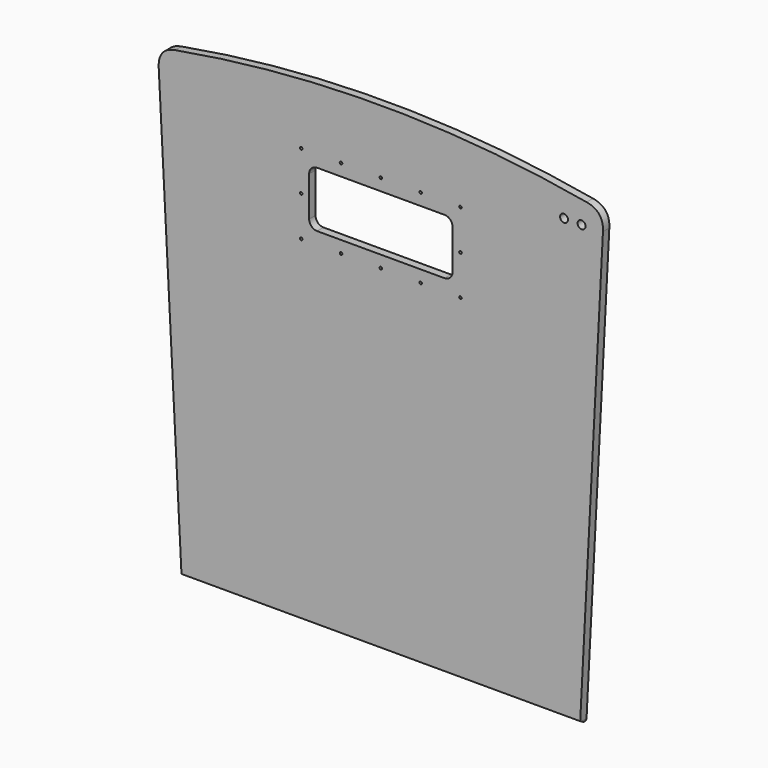
from build123d import *

# Parameters (mm, degrees)
F1_DEPTH    = 10
F2_W        = 180
F2_H        = 70
F3_DEPTH    = 10.001
F4_T1_DEPTH = 120.3455223822
F5_R        = 5
F6_T1_DEPTH = 541.5885597996
F7_R        = 10
F9_D        = 3.2
F9_DEPTH    = 6
F9_TIP      = 0.9613769904
F11_D       = 10


# Not quite as in the source:
# - a fillet or chamfer that OpenCascade refuses, or shapes differently, is made with other operations: its cross-section is extruded or revolved along the edge and cut away or added


with BuildPart() as f1:
    # F0 (on Front) → F1 (new body)
    with BuildSketch(Plane.XZ):
        with BuildLine():
            Line((-30, 578), (0, 0))
            Line((0, 0), (500, 0))
            Line((500, 0), (530, 578))
            ThreePointArc((530, 578), (250, 605), (-30, 578))
        make_face()
    extrude(amount=F1_DEPTH)

    # F2 (on face) → F3 (cut, through all)
    with BuildSketch(Plane.XZ.offset(10)):
        with Locations((250, 475)):
            Rectangle(F2_W, F2_H)
    extrude(amount=-F3_DEPTH, mode=Mode.SUBTRACT)

    # F4: fillet of radius 25 on 2 edges, made by hand

    # F4_s2 → F4_t1 (cut)
    with BuildSketch(Plane.XZ.offset(-55.1727611911)):
        with BuildLine():
            add(Edge.make_bspline(
                [(-28.865884536, 556.1493753933), (-30.0086821523, 578.1672761351), (-8.3063912994, 582.0537283993)],
                knots=[0, 0, 0, 1, 1, 1], degree=2, weights=[1, 1, 1]))
            ThreePointArc((-8.3063912994, 582.0537283993), (-19.1608272147, 580.0677046728), (-30, 578))
            Line((-30, 578), (-28.865884536, 556.1493753933))
        make_face()
        with BuildLine():
            add(Edge.make_bspline(
                [(508.3063912994, 582.0537283993), (530.0086821523, 578.1672761351), (528.865884536, 556.1493753933)],
                knots=[0, 0, 0, 1, 1, 1], degree=2, weights=[1, 1, 1]))
            Line((528.865884536, 556.1493753933), (530, 578))
            ThreePointArc((530, 578), (519.1608272147, 580.0677046728), (508.3063912994, 582.0537283993))
        make_face()
    extrude(amount=F4_T1_DEPTH, mode=Mode.SUBTRACT)

    # F5
    f5_edges = [f1.edges().sort_by_distance(p)[0] for p in [
        (500, -5, 0),
        (0, -5, 0),
    ]]
    fillet(f5_edges, radius=F5_R)

    # F6: chamfer of 5.7 x 9.8726896031 on 1 edges, made by hand

    # F6_s2 → F6_t1 (cut)
    with BuildSketch(Plane.YZ.offset(-20.7942798998)):
        Polygon((-10, 5.7), (-0.1273103969, 0), (-10, 0), align=None)
    extrude(amount=F6_T1_DEPTH, mode=Mode.SUBTRACT)

    # F7
    f7_edges = [f1.edges().sort_by_distance(p)[0] for p in [
        (340, -5, 510),
        (160, -5, 510),
        (160, -5, 440),
        (340, -5, 440),
    ]]
    fillet(f7_edges, radius=F7_R)

    # F9
    with Locations(Plane.XZ.offset(10)):
        with Locations((150, 525), (200, 525), (250, 525), (250, 425), (200, 425), (150, 425), (150, 475), (350, 525), (350, 475), (350, 425), (300, 425), (300, 525)):
            Hole(F9_D / 2, depth=F9_DEPTH)
            with Locations((0, 0, -(F9_DEPTH + F9_TIP / 2))):  # 118° drill point
                Cone(0, F9_D / 2, F9_TIP, mode=Mode.SUBTRACT)

    # F11 (through all)
    with Locations(Plane.XZ.offset(10)):
        with Locations((480, 555), (502, 555)):
            Hole(F11_D / 2)


solid = f1.part
